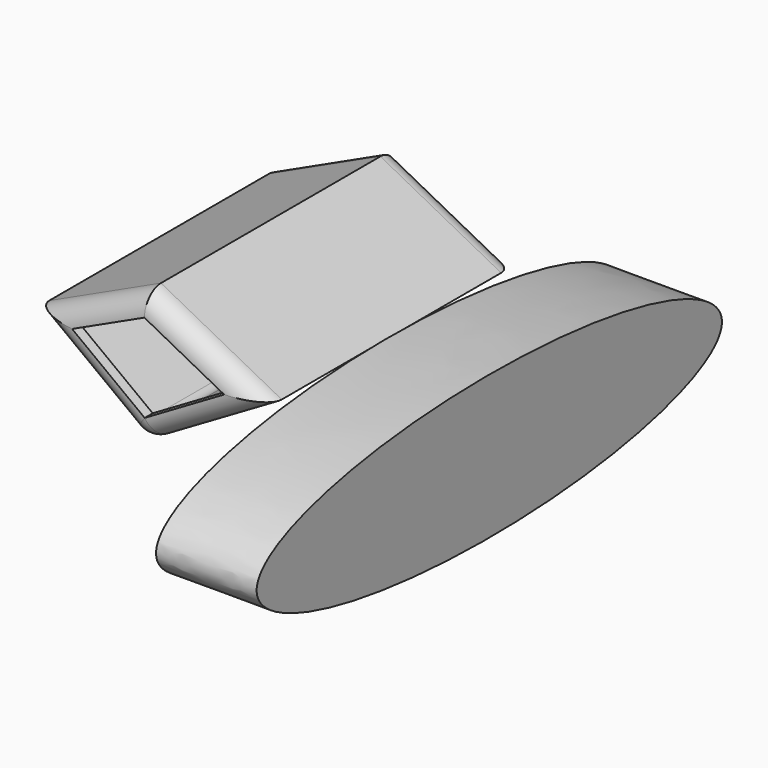
from build123d import *

# Parameters (mm, degrees)
F1_DEPTH = 25.4
F3_DEPTH = 25.4
F4_DEPTH = 40.5853167176
F5_DEPTH = 13.4420320392
F6_R     = 5.08
F8_DEPTH = 18.0026832968
F9_T     = -2.54


# Not quite as in the source:
# - a shell that OpenCascade refuses in one call is made with other operations: the cavity is built on its own and cut out


with BuildPart() as f1:
    # F0 (on Right) → F1 (new body)
    with BuildSketch(Plane.YZ):
        with BuildLine():
            add(Edge.make_bspline(
                [(73.4398514032, 0), (73.4398514032, 31.4291412197), (-36.7199257016, 15.7145706098), (-146.8797028065, 0), (-36.7199257016, -15.7145706098), (73.4398514032, -31.4291412197), (73.4398514032, 0)],
                knots=[0, 0, 0, 2.0943951024, 2.0943951024, 4.1887902048, 4.1887902048, 6.2831853072, 6.2831853072, 6.2831853072], degree=2, weights=[1, 0.5, 1, 0.5, 1, 0.5, 1]))
        make_face()
    extrude(amount=F1_DEPTH)


with BuildPart() as f3:
    # F2 (on Front) → F3 (new body)
    with BuildSketch(Plane.XZ):
        Polygon((-30.9111475945, 0), (0, 18.0487856269), (-30.4962322116, 34.0229794383), (-58.7103962898, 20.9531858563), align=None)
    extrude(amount=F3_DEPTH)

    # F4 (add): a face of the model
    f4_faces = [f3.faces().sort_by_distance(p)[0] for p in [
        (-29.8150802382, 0, 17.8195988586),
    ]]
    extrude(f4_faces, amount=F4_DEPTH)

    # F5 (add): a face of the model
    f5_faces = [f3.faces().sort_by_distance(p)[0] for p in [
        (-29.8150802382, -25.4, 17.8195988586),
    ]]
    extrude(f5_faces, amount=F5_DEPTH)

    # F6
    f6_edges = [f3.edges().sort_by_distance(p)[0] for p in [
        (-15.248116, -38.842032, 26.035883),
        (-44.603314, -38.842032, 27.488083),
        (-30.911148, 0.871642, 0),
        (-15.455574, -38.842032, 9.024393),
        (-44.810772, -38.842032, 10.476593),
        (-15.248116, 40.585317, 26.035883),
        (-44.603314, 40.585317, 27.488083),
        (-15.455574, 40.585317, 9.024393),
        (-44.810772, 40.585317, 10.476593),
    ]]
    fillet(f6_edges, radius=F6_R)

    # F7 (on face) → F8 (join)
    with BuildSketch(Plane.XZ.offset(38.8420320392)):
        Polygon((-48.8827081385, 19.9071354088), (-39.7179437035, 12.9993583448), (-20.5204627354, 11.9496086934), (-10.4877462022, 17.807636106), (-30.6341607446, 28.3605046792), align=None)
        Polygon((-20.5204627354, 11.9496086934), (-39.7179437035, 12.9993583448), (-30.5531792686, 6.0915812808), align=None)
    extrude(amount=-F8_DEPTH)

    # F9: a shell. OpenCascade refuses it in one call, so the cavity is built on its own and cut out:
    # the body offset inwards by the wall thickness, plus a prism from it out through each open face.
    f9_core = offset(f3.part, amount=F9_T, mode=Mode.PRIVATE)
    f9_exits = [f9_core.faces().sort_by_distance(p)[0] for p in [
        (-29.986003, -36.302032, 17.753154),
    ]]
    add(f9_core, mode=Mode.SUBTRACT)
    extrude(f9_exits, amount=-F9_T, mode=Mode.SUBTRACT)


solid = Compound([f1.part, f3.part])
